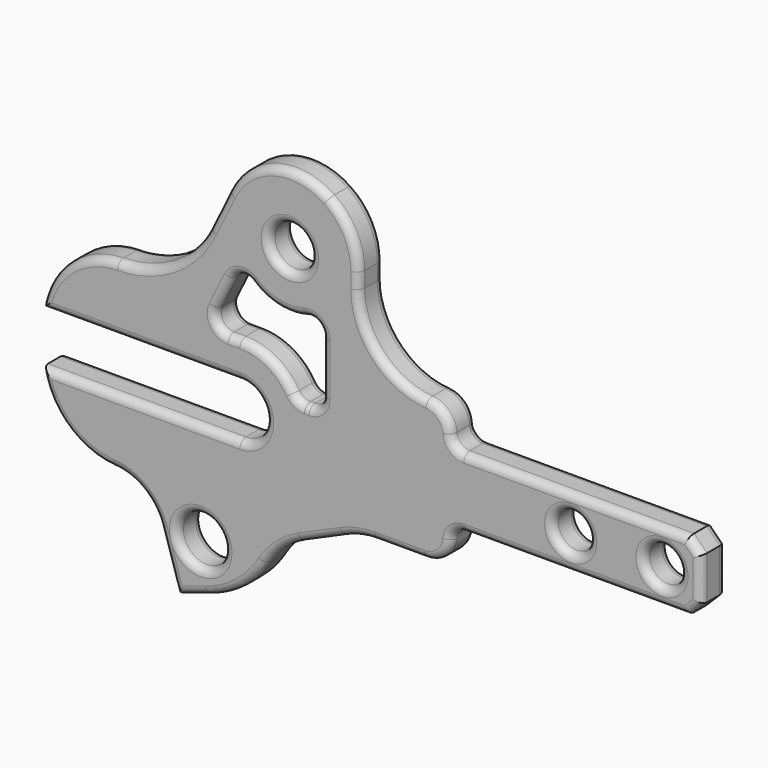
from build123d import *

# Parameters (mm, degrees)
F0_R        = 4.5
F0_R_2      = 3.5
F0_R_3      = 4
F1_DEPTH    = 3
F2_T1_DEPTH = 80.0337760755
F3_R        = 20
F4_R        = 14
F5_R        = 5
F6_SIZE     = 2.5
F7_R        = 15
F8_R        = 20
F9_R        = 10
F10_R       = 2.5
F11_R       = 2.5
F12_R       = 1.49999


# Not quite as in the source:
# - a fillet or chamfer that OpenCascade refuses, or shapes differently, is made with other operations: its cross-section is extruded or revolved along the edge and cut away or added
# - a fillet or chamfer is up to 0.001 mm smaller than in the source, because OpenCascade refuses the exact size
# - ends of sketch curves that miss each other by under 0.0002 mm in the source are joined


with BuildPart() as f1:
    # F0 (on Front) → F1 (new body, symmetric)
    with BuildSketch(Plane.XZ):
        with BuildLine():
            ThreePointArc((0, 5), (5, 0), (0, -5))
            Line((0, -5), (-38, -5))
            Line((-38, -5), (-38, -17.6))
            Line((-38, -17.6), (-17.5184067676, -17.6))
            Line((-17.5184067676, -17.6), (-12.0535889556, -35.0600581259))
            Line((-12.0535889556, -35.0600581259), (2.4043341203, -30.5348775693))
            Line((2.4043341203, -30.5348775693), (6.0098162888, -20.9202609368))
            Line((6.0098162888, -20.9202609368), (22.8, -13.5334727884))
            Line((22.8, -13.5334727884), (40.5, -13.5334727884))
            Line((40.5, -13.5334727884), (40.5, -6.65))
            Line((40.5, -6.65), (88.5, -6.65))
            Line((88.5, -6.65), (88.5, 6.65))
            Line((88.5, 6.65), (40.5, 6.65))
            Line((40.5, 6.65), (40.5, 13.5334727884))
            Line((40.5, 13.5334727884), (22.8, 13.5334727884))
            Line((22.8, 13.5334727884), (22.8, 30.5325201458))
            ThreePointArc((22.8, 30.5325201458), (21.2721913634, 36.696929994), (17.0424320036, 41.4343642959))
            Line((17.0424320036, 41.4343642959), (17.0041085128, 41.4604283231))
            ThreePointArc((17.0041085128, 41.4604283231), (6.2010093498, 43.2511126057), (-2.2364375725, 36.2709799418))
            Line((-2.2364375725, 36.2709799418), (-11.3, 17.6))
            Line((-11.3, 17.6), (-38, 17.6))
            Line((-38, 17.6), (-38, 5))
            Line((-38, 5), (0, 5))
        make_face()
        with Locations((-7.5, -24.5)):
            Circle(F0_R, mode=Mode.SUBTRACT)
        with Locations((63.5, 0)):
            Circle(F0_R_2, mode=Mode.SUBTRACT)
        with Locations((81, 0)):
            Circle(F0_R_2, mode=Mode.SUBTRACT)
        with BuildLine():
            Line((0, 12), (-6.2372614463, 12))
            Line((-6.2372614463, 12), (0.0821313233, 25.0179779298))
            ThreePointArc((0.0821313233, 25.0179779298), (7.1625129229, 19.8059803147), (15.8, 21.4462667926))
            Line((15.8, 21.4462667926), (15.8, 5))
            Line((15.8, 5), (10.9087121146, 5))
            ThreePointArc((10.9087121146, 5), (6.4807406984, 10.0995049384), (0, 12))
        make_face(mode=Mode.SUBTRACT)
        with Locations((9.6, 30.5325201458)):
            Circle(F0_R_3, mode=Mode.SUBTRACT)
    extrude(amount=F1_DEPTH, both=True)

    # F2: fillet of radius 15 on 2 edges, made by hand

    # F2_s2 → F2_t1 (cut)
    with BuildSketch(Plane.XZ.offset(-40.0168880378)):
        with BuildLine():
            ThreePointArc((-38, 5), (-32.9143558325, 14.0236596588), (-23.1932447849, 17.6))
            Line((-23.1932447849, 17.6), (-38, 17.6))
            Line((-38, 17.6), (-38, 5))
        make_face()
        with BuildLine():
            ThreePointArc((-23.1932447849, -17.6), (-32.9143558325, -14.0236596588), (-38, -5))
            Line((-38, -5), (-38, -17.6))
            Line((-38, -17.6), (-23.1932447849, -17.6))
        make_face()
    extrude(amount=F2_T1_DEPTH, mode=Mode.SUBTRACT)

    # F3
    f3_edges = [f1.edges().sort_by_distance(p)[0] for p in [
        (-11.3, 0, 17.6),
    ]]
    fillet(f3_edges, radius=F3_R)

    # F4
    f4_edges = [f1.edges().sort_by_distance(p)[0] for p in [
        (22.8, 0, 13.533473),
    ]]
    fillet(f4_edges, radius=F4_R)

    # F5
    f5_edges = [f1.edges().sort_by_distance(p)[0] for p in [
        (40.5, 0, -13.533473),
        (40.5, 0, 13.533473),
    ]]
    fillet(f5_edges, radius=F5_R)

    # F6
    f6_edges = [f1.edges().sort_by_distance(p)[0] for p in [
        (88.5, 0, 6.65),
        (88.5, 0, -6.65),
    ]]
    chamfer(f6_edges, length=F6_SIZE)

    # F7
    f7_edges = [f1.edges().sort_by_distance(p)[0] for p in [
        (22.8, 0, -13.533473),
        (6.009816, 0, -20.920261),
    ]]
    fillet(f7_edges, radius=F7_R)

    # F8
    f8_edges = [f1.edges().sort_by_distance(p)[0] for p in [
        (2.404334, 0, -30.534878),
    ]]
    fillet(f8_edges, radius=F8_R)

    # F9
    f9_edges = [f1.edges().sort_by_distance(p)[0] for p in [
        (-17.518407, 0, -17.6),
    ]]
    fillet(f9_edges, radius=F9_R)

    # F10
    f10_edges = [f1.edges().sort_by_distance(p)[0] for p in [
        (40.5, 0, 6.65),
        (40.5, 0, -6.65),
    ]]
    fillet(f10_edges, radius=F10_R)

    # F11
    f11_edges = [f1.edges().sort_by_distance(p)[0] for p in [
        (0.082131, 0, 25.017978),
        (15.8, 0, 21.446267),
        (-6.237261, 0, 12),
        (10.908712, 0, 5),
        (15.8, 0, 5),
    ]]
    fillet(f11_edges, radius=F11_R)

    # F12 (radius 1.5 in the source; OpenCascade refuses exactly that, so slightly less here)
    f12_edges = [f1.edges().sort_by_distance(p)[0] for p in [
        (7.154424, -3, 19.807822),
        (0.149426, -3, 22.888878),
        (14.80616, -3, 19.544819),
        (-3.052692, -3, 18.560228),
        (15.8, -3, 12.524727),
        (-4.363569, -3, 13.173234),
        (15.067767, -3, 5.732233),
        (-1.12234, -3, 12),
        (12.854837, -3, 5),
        (5.895644, -3, 10.45186),
        (11.181414, -3, 5.322529),
        (38.887101, -3, -12.211454),
        (41.281066, -3, -7.311009),
        (30.726871, -3, -13.533473),
        (64.487308, -3, -6.65),
        (22.867476, -3, -13.854407),
        (87.25, -3, -5.4),
        (15.854166, -3, -16.589271),
        (88.5, -3, 0),
        (7.90732, -3, -20.860914),
        (87.25, -3, 5.4),
        (0.175289, -3, -29.856272),
        (64.489078, -3, 6.65),
        (-9.144419, -3, -34.149518),
        (41.279137, -3, 7.316061),
        (-13.697467, -3, -29.807879),
        (39.021601, -3, 12.127411),
        (-18.693862, -3, -19.689546),
        (26.567441, -3, 17.978645),
        (-33.295484, -3, -13.688046),
        (22.8, -3, 29.032996),
        (-19, -3, -5),
        (21.272191, -3, 36.69693),
        (5, -3, 0),
        (17.02327, -3, 41.447396),
        (-19, -3, 5),
        (6.201027, -3, 43.251117),
        (-33.017226, -3, 13.935317),
        (-4.035153, -3, 32.565617),
        (-13.059071, -3, 20.739808),
        (-12, -3, -24.5),
        (60, -3, 0),
        (77.5, -3, 0),
        (5.6, -3, 30.53252),
        (7.154424, 3, 19.807822),
        (0.149426, 3, 22.888878),
        (14.80616, 3, 19.544819),
        (-3.052692, 3, 18.560228),
        (15.8, 3, 12.524727),
        (-4.363569, 3, 13.173234),
        (15.067767, 3, 5.732233),
        (-1.12234, 3, 12),
        (12.854837, 3, 5),
        (5.895644, 3, 10.45186),
        (11.181414, 3, 5.322529),
        (38.887101, 3, -12.211454),
        (41.281066, 3, -7.311009),
        (30.726871, 3, -13.533473),
        (64.487308, 3, -6.65),
        (22.867476, 3, -13.854407),
        (87.25, 3, -5.4),
        (15.854166, 3, -16.589271),
        (88.5, 3, 0),
        (7.90732, 3, -20.860914),
        (87.25, 3, 5.4),
        (0.175289, 3, -29.856272),
        (64.489078, 3, 6.65),
        (-9.144419, 3, -34.149518),
        (41.279137, 3, 7.316061),
        (-13.697467, 3, -29.807879),
        (39.021601, 3, 12.127411),
        (-18.693862, 3, -19.689546),
        (26.567441, 3, 17.978645),
        (-33.295484, 3, -13.688046),
        (22.8, 3, 29.032996),
        (-19, 3, -5),
        (21.272191, 3, 36.69693),
        (5, 3, 0),
        (17.02327, 3, 41.447396),
        (-19, 3, 5),
        (6.201027, 3, 43.251117),
        (-33.017226, 3, 13.935317),
        (-4.035153, 3, 32.565617),
        (-13.059071, 3, 20.739808),
        (-12, 3, -24.5),
        (60, 3, 0),
        (77.5, 3, 0),
        (5.6, 3, 30.53252),
    ]]
    fillet(f12_edges, radius=F12_R)


solid = f1.part
